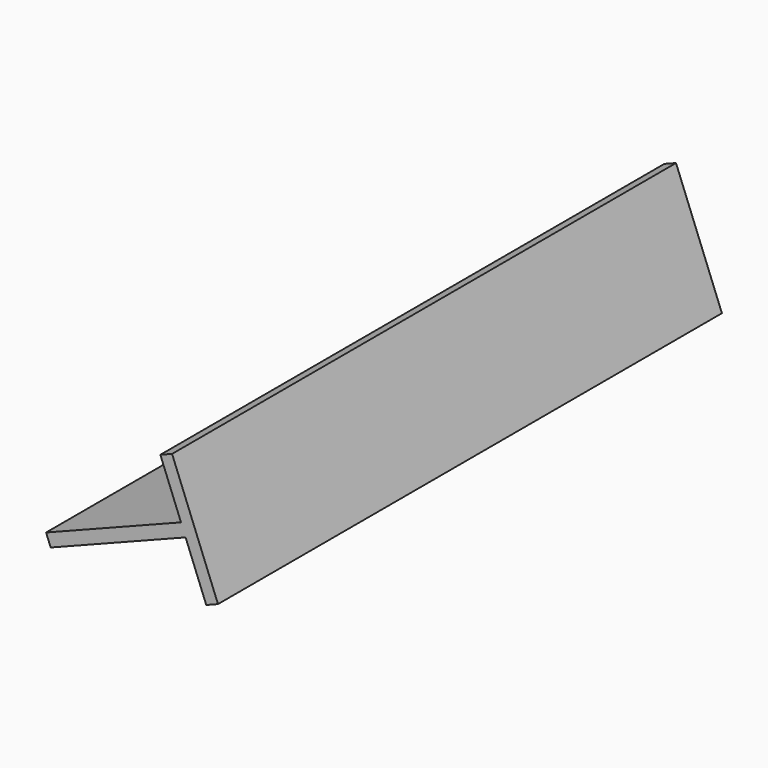
from build123d import *

# Parameters (mm, degrees)
F1_DEPTH = 400


# Not quite as in the source:
# - the program builds the solid bodies; features that only make, move or delete a surface that nothing else refers to are left out


with BuildPart() as f1:
    # F0 (on Front) → F1 (new body)
    with BuildSketch(Plane.XZ):
        Polygon((-80.0059014217, 7.4499422376), (-77.090706633, 0), (8.5836290999, 33.5247400694), (21.7020056488, 0), (29.1519478864, 2.9151947886), (0, 77.4146171651), (-7.4499422376, 74.4994223765), (5.6684343113, 40.9746823071), align=None)
    extrude(amount=-F1_DEPTH)


solid = f1.part
